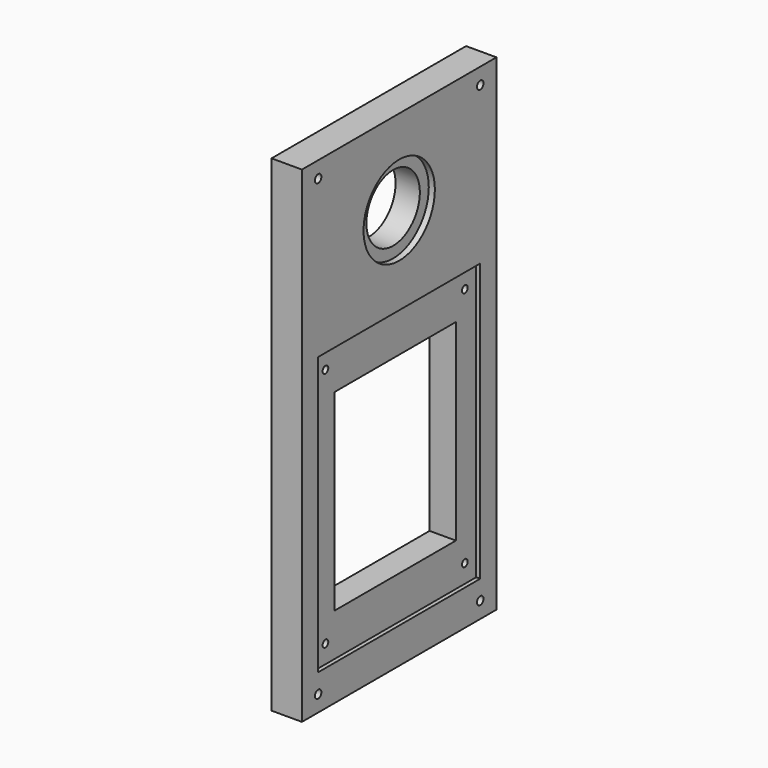
from build123d import *

# Parameters (mm, degrees)
F0_W     = 120
F0_H     = 240
F0_R     = 2
F0_R_2   = 22
F1_DEPTH = 15
F0_R_3   = 16.5
F2_DEPTH = 12
F0_R_4   = 1.75
F0_W_2   = 75
F0_H_2   = 95
F3_DEPTH = 13


# Not quite as in the source:
# - a feature names something its author has since deleted; it is built from what else it names


with BuildPart() as f1:
    # F0 (on Right) → F1 (new body)
    with BuildSketch(Plane.YZ):
        with Locations((-10.4347826087, 0)):
            Rectangle(F0_W, F0_H)
        with Locations((-60.4347826087, -112)):
            Circle(F0_R, mode=Mode.SUBTRACT)
        with Locations((39.5652173913, -112)):
            Circle(F0_R, mode=Mode.SUBTRACT)
        Polygon((-60.4347826087, -102.5), (-60.4347826087, 25.4482906163), (-60.4347826087, 34.5), (39.5652173913, 34.5), (39.5652173913, 25.4482906163), (39.5652173913, -102.5), align=None, mode=Mode.SUBTRACT)
        with Locations((-60.4347826087, 112)):
            Circle(F0_R, mode=Mode.SUBTRACT)
        with Locations((-10.4347826087, 78)):
            Circle(F0_R_2, mode=Mode.SUBTRACT)
        with Locations((39.5652173913, 112.0000034571)):
            Circle(F0_R, mode=Mode.SUBTRACT)
    extrude(amount=F1_DEPTH)

    # F0 (on Right) → F2 (join)
    with BuildSketch(Plane.YZ):
        with Locations((-10.4347826087, 78)):
            Circle(F0_R_2)
        with Locations((-10.4347826087, 78)):
            Circle(F0_R_3, mode=Mode.SUBTRACT)
    extrude(amount=F2_DEPTH)

    # F0 (on Right) → F3 (join)
    with BuildSketch(Plane.YZ):
        Polygon((-60.4347826087, 34.5), (-60.4347826087, 25.4482906163), (-60.4347826087, -102.5), (39.5652173913, -102.5), (39.5652173913, 25.4482906163), (39.5652173913, 34.5), align=None)
        with Locations((-53.4347826087, -93.5)):
            Circle(F0_R_4, mode=Mode.SUBTRACT)
        with Locations((32.5652173913, -93.5)):
            Circle(F0_R_4, mode=Mode.SUBTRACT)
        with Locations((-10.4347826087, -34)):
            Rectangle(F0_W_2, F0_H_2, mode=Mode.SUBTRACT)
        with Locations((-53.4347826087, 25.5)):
            Circle(F0_R_4, mode=Mode.SUBTRACT)
        with Locations((32.5652173913, 25.5)):
            Circle(F0_R_4, mode=Mode.SUBTRACT)
    extrude(amount=F3_DEPTH)


solid = f1.part
